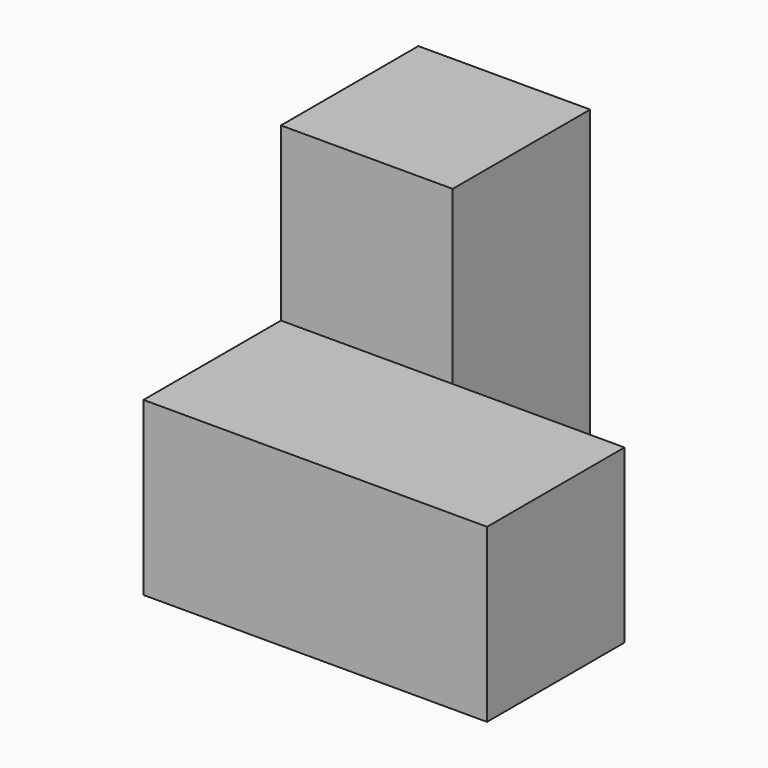
from build123d import *

# Parameters (mm, degrees)
F1_W     = 152.4
F1_H     = 76.2
F2_DEPTH = 76.2
F3_W     = 76.2
F3_H     = 76.2
F4_DEPTH = 76.2
F5_W     = 76.2
F5_H     = 76.2
F6_DEPTH = 76.2


# Not quite as in the source:
# - a variable given as a bare number and used for a length is read in inches; the dataset says mm whatever the document's units were


with BuildPart() as f2:
    # F1 (on Front) → F2 (new body)
    with BuildSketch(Plane.XZ):
        with Locations((0, -5.0575301152)):
            Rectangle(F1_W, F1_H)
    extrude(amount=F2_DEPTH)

    # F3 (on face) → F4 (join)
    with BuildSketch(Plane(origin=(0, 0, 0), x_dir=(-1, 0, 0), z_dir=(0, 1, 0))):
        with Locations((38.1, -5.0575301152)):
            Rectangle(F3_W, F3_H)
    extrude(amount=F4_DEPTH)

    # F5 (on face) → F6 (join)
    with BuildSketch(Plane.XY.offset(33.0424698848)):
        with Locations((-38.1, 38.1)):
            Rectangle(F5_W, F5_H)
    extrude(amount=F6_DEPTH)


solid = f2.part
